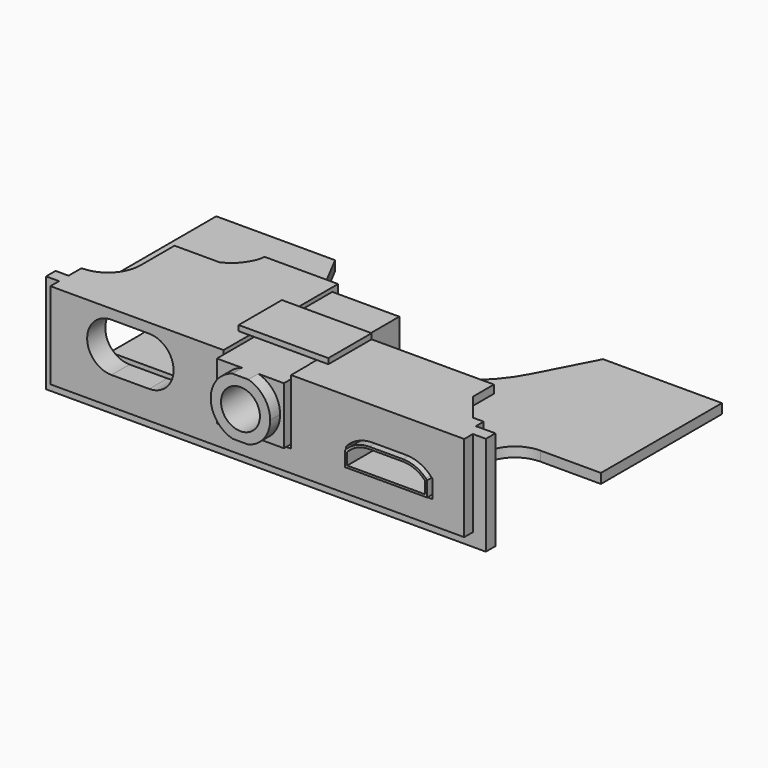
from build123d import *

# Parameters (mm, degrees)
F0_W      = 46.8
F0_H      = 24
F1_DEPTH  = 0.9
F3_DEPTH  = 25
F4_R      = 1
F5_R      = 4
F6_R      = 0.75
F7_DEPTH  = 25
F8_R      = 1.075
F9_DEPTH  = 25
F10_W     = 7.6
F10_H     = 5.1
F11_DEPTH = 2.4
F12_SIZE  = 1
F13_R     = 3
F15_DEPTH = 3
F16_W     = 6.2
F16_H     = 14.5
F17_DEPTH = 5.3
F18_R     = 1.8
F19_DEPTH = 14.5
F20_R     = 1.8
F21_DEPTH = 1.15
F24_DEPTH = 1
F26_DEPTH = 1.1
F28_DEPTH = 0.75
F29_W     = 8.3
F29_H     = 5
F30_DEPTH = 0.5
F32_DEPTH = 0.75
F34_DEPTH = 25


with BuildPart() as f1:
    # F0 (on Top) → F1 (new body)
    with BuildSketch(Plane.XY):
        Rectangle(F0_W, F0_H)
    extrude(amount=F1_DEPTH)

    # F2 (on face) → F3 (cut)
    with BuildSketch(Plane.XY.offset(0.9)):
        Polygon((-16.1, -2), (-23.4, -2), (-23.4, -12), (-16.1, -12), (-4.6, -12), (-4.6, -9.4), (-16.1, -9.4), align=None)
        with BuildLine():
            Line((-12.4, 12), (-9.7580645161, 6.9225816699))
            ThreePointArc((-9.7580645161, 6.9225816699), (0, 1), (9.7580645161, 6.9225816699))
            Line((9.7580645161, 6.9225816699), (12.4, 12))
            Line((12.4, 12), (-12.4, 12))
        make_face()
        with BuildLine():
            Line((17.1, -12), (23.4, -12))
            Line((23.4, -12), (23.4, -2))
            Line((23.4, -2), (17.7911840902, -2))
            ThreePointArc((17.7911840902, -2), (14.8706646396, -4.5931467489), (17.1, -7.8))
            Line((17.1, -7.8), (17.1, -12))
        make_face()
    extrude(amount=-F3_DEPTH, mode=Mode.SUBTRACT)

    # F4
    f4_edges = [f1.edges().sort_by_distance(p)[0] for p in [
        (-4.6, -9.4, 0.45),
    ]]
    fillet(f4_edges, radius=F4_R)

    # F5
    f5_edges = [f1.edges().sort_by_distance(p)[0] for p in [
        (-16.1, -2, 0.45),
    ]]
    fillet(f5_edges, radius=F5_R)

    # F6 (on face) → F7 (cut)
    with BuildSketch(Plane.XY.offset(0.9)):
        with Locations((-8.5, 2.75)):
            Circle(F6_R)
        with Locations((8.5, 2.75)):
            Circle(F6_R)
    extrude(amount=-F7_DEPTH, mode=Mode.SUBTRACT)

    # F8 (on face) → F9 (cut)
    with BuildSketch(Plane.XY.offset(0.9)):
        with Locations((7.825, -5.025)):
            Circle(F8_R)
    extrude(amount=-F9_DEPTH, mode=Mode.SUBTRACT)


with BuildPart() as f11:
    # F10 (on face) → F11 (new body)
    with BuildSketch(Plane.XY.offset(0.9)):
        with Locations((12.2, -10.3)):
            Rectangle(F10_W, F10_H)
    extrude(amount=F11_DEPTH)

    # F12
    f12_edges = [f11.edges().sort_by_distance(p)[0] for p in [
        (8.4, -10.3, 3.3),
        (16, -10.3, 3.3),
    ]]
    chamfer(f12_edges, length=F12_SIZE)

    # F13
    f13_edges = [f11.edges().sort_by_distance(p)[0] for p in [
        (9.4, -10.3, 3.3),
        (15, -10.3, 3.3),
    ]]
    fillet(f13_edges, radius=F13_R)

    # F14 (on face) → F15 (cut)
    with BuildSketch(Plane.XZ.offset(12.85)):
        with BuildLine():
            Line((13.7573593129, 3.1), (10.6426406871, 3.1))
            ThreePointArc((10.6426406871, 3.1), (9.5296016157, 2.8692691618), (8.6, 2.2151028754))
            Line((8.6, 2.2151028754), (8.6, 1.1))
            Line((8.6, 1.1), (15.8, 1.1))
            Line((15.8, 1.1), (15.8, 2.2151028754))
            ThreePointArc((15.8, 2.2151028754), (14.8703983843, 2.8692691618), (13.7573593129, 3.1))
        make_face()
    extrude(amount=-F15_DEPTH, mode=Mode.SUBTRACT)


with BuildPart() as f17:
    # F16 (on face) → F17 (new body)
    with BuildSketch(Plane.XY.offset(0.9)):
        with Locations((0, -7.2)):
            Rectangle(F16_W, F16_H)
    extrude(amount=F17_DEPTH)

    # F18 (on face) → F19 (cut, through all)
    with BuildSketch(Plane.XZ.offset(14.45)):
        with Locations((0, 3.55)):
            Circle(F18_R)
    extrude(amount=-F19_DEPTH, mode=Mode.SUBTRACT)

    # F20 (on face) → F21 (cut)
    with BuildSketch(Plane.XZ.offset(14.45)):
        with Locations((0, 3.55)):
            Circle(F20_R)
        with BuildLine():
            Line((-0.7348469228, 6.2), (0.7348469228, 6.2))
            ThreePointArc((0.7348469228, 6.2), (0, 6.3), (-0.7348469228, 6.2))
        make_face()
        with BuildLine():
            ThreePointArc((-0.7348469228, 0.9), (0, 0.8), (0.7348469228, 0.9))
            Line((0.7348469228, 0.9), (-0.7348469228, 0.9))
        make_face()
        with BuildLine():
            ThreePointArc((-0.7348469228, 0.9), (-2.75, 3.55), (-0.7348469228, 6.2))
            Line((-0.7348469228, 6.2), (-3.1, 6.2))
            Line((-3.1, 6.2), (-3.1, 0.9))
            Line((-3.1, 0.9), (-0.7348469228, 0.9))
        make_face()
        with BuildLine():
            ThreePointArc((0.7348469228, 6.2), (2.1889870988, 5.2145826748), (2.75, 3.55))
            ThreePointArc((2.75, 3.55), (2.1889870988, 1.8854173252), (0.7348469228, 0.9))
            Line((0.7348469228, 0.9), (3.1, 0.9))
            Line((3.1, 0.9), (3.1, 6.2))
            Line((3.1, 6.2), (0.7348469228, 6.2))
        make_face()
    extrude(amount=-F21_DEPTH, mode=Mode.SUBTRACT)


with BuildPart() as f24:
    # F23 (on offset) → F24 (new body)
    with BuildSketch(Plane(origin=(0, -12.5, 0), x_dir=(-1, 0, 0), z_dir=(0, 1, 0))):
        Polygon((19.15, -1.45), (19.15, 6.55), (3.125, 6.55), (3.125, 0.55), (-3.125, 0.55), (-3.125, 6.55), (-19.15, 6.55), (-19.15, -1.45), align=None)
        with BuildLine():
            Line((-16.2, 0.7), (-16.2, 2.3672461086))
            ThreePointArc((-16.2, 2.3672461086), (-15.1036156875, 3.2030318245), (-13.7573593129, 3.5))
            Line((-13.7573593129, 3.5), (-10.6426406871, 3.5))
            ThreePointArc((-10.6426406871, 3.5), (-9.2963843125, 3.2030318245), (-8.2, 2.3672461086))
            Line((-8.2, 2.3672461086), (-8.2, 0.7))
            Line((-8.2, 0.7), (-16.2, 0.7))
        make_face(mode=Mode.SUBTRACT)
    extrude(amount=F24_DEPTH)

    # F25 (on face) → F26 (join)
    with BuildSketch(Plane(origin=(0, -11.5, 0), x_dir=(-1, 0, 0), z_dir=(0, 1, 0))):
        Polygon((20.35, -2.65), (20.35, 6.55), (3.125, 6.55), (3.125, 0.55), (-3.125, 0.55), (-3.125, 6.55), (-20.35, 6.55), (-20.35, -2.65), align=None)
        with BuildLine():
            Line((-13.7573593129, 3.5), (-10.6426406871, 3.5))
            ThreePointArc((-10.6426406871, 3.5), (-9.2963843125, 3.2030318245), (-8.2, 2.3672461086))
            Line((-8.2, 2.3672461086), (-8.2, 0.7))
            Line((-8.2, 0.7), (-16.2, 0.7))
            Line((-16.2, 0.7), (-16.2, 2.3672461086))
            ThreePointArc((-16.2, 2.3672461086), (-15.1036156875, 3.2030318245), (-13.7573593129, 3.5))
        make_face(mode=Mode.SUBTRACT)
    extrude(amount=F26_DEPTH)

    # F27 (on face) → F28 (join)
    with BuildSketch(Plane.XY.offset(6.55)):
        with BuildLine():
            Line((-19.15, -10.4), (-3.125, -10.4))
            Line((-3.125, -10.4), (-3.125, 0.75))
            Line((-3.125, 0.75), (-9.925, 0.75))
            add(Edge.make_bspline(
                [(-11.85, -1.95), (-10.9984157607, -1.39684428), (-10.6160626022, -0.9492889302), (-9.9995483018, 0), (-9.925, 0.75)],
                knots=[0, 0, 0, 0, 0.5017533344, 1, 1, 1, 1], degree=3))
            Line((-11.85, -1.95), (-16.1, -1.95))
            Line((-16.1, -1.95), (-16.1, -5.9004166956))
            ThreePointArc((-16.1, -5.9004166956), (-16.9610750364, -8.0039850924), (-19.05, -8.9))
            ThreePointArc((-19.05, -8.9), (-19.1, -8.9004166956), (-19.15, -8.9))
            Line((-19.15, -8.9), (-19.15, -10.4))
        make_face()
        with BuildLine():
            Line((-19.05, -8.9), (-19.15, -8.9))
            ThreePointArc((-19.15, -8.9), (-19.1, -8.9004166956), (-19.05, -8.9))
        make_face()
    extrude(amount=-F28_DEPTH)

    # F29 (on face) → F30 (join)
    with BuildSketch(Plane.XY.offset(6.55)):
        with Locations((0.025, -7)):
            Rectangle(F29_W, F29_H)
    extrude(amount=F30_DEPTH)

    # F31 (on face) → F32 (join, through all)
    with BuildSketch(Plane.XY.offset(6.55)):
        Polygon((15.5, -4.5), (3.1, -4.5), (3.1, -10.4), (15.5, -10.4), (18.55, -10.4), (18.55, -9.5), (17.55, -9.5), (15.5, -6.9), align=None)
    extrude(amount=-F32_DEPTH)

    # F33 (on face) → F34 (cut)
    with BuildSketch(Plane.XZ.offset(12.5)):
        with BuildLine():
            Line((-10, 5.65), (-13.5, 5.65))
            ThreePointArc((-13.5, 5.65), (-15.75, 3.4), (-13.5, 1.15))
            Line((-13.5, 1.15), (-10, 1.15))
            ThreePointArc((-10, 1.15), (-7.75, 3.4), (-10, 5.65))
        make_face()
    extrude(amount=-F34_DEPTH, mode=Mode.SUBTRACT)


solid = Compound([f1.part, f11.part, f17.part, f24.part])
